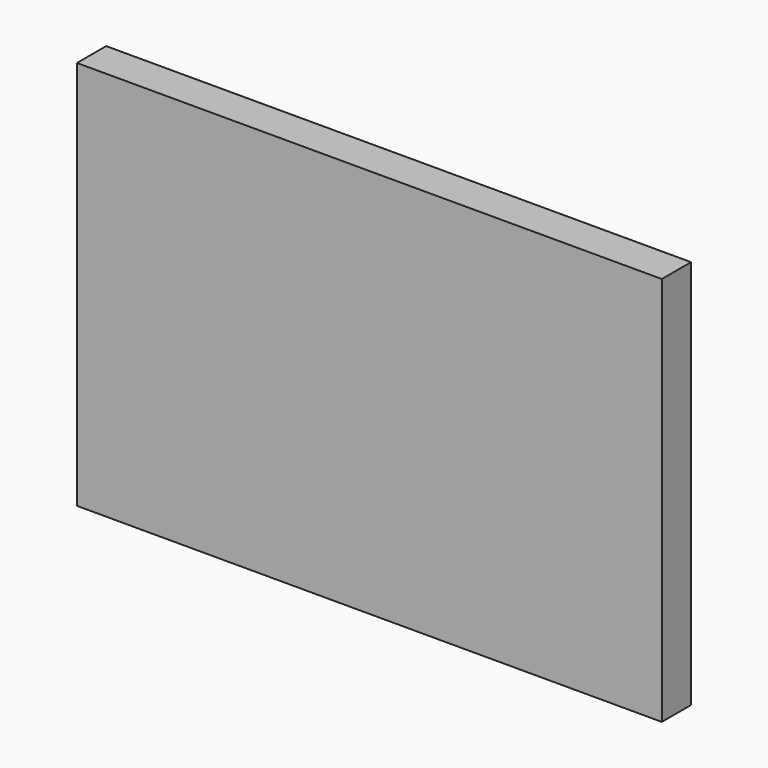
from build123d import *

# Parameters (mm, degrees)
F0_W     = 76.2
F0_H     = 50.8
F1_DEPTH = 4.7625


# Not quite as in the source:
# - a length typed as a fraction of an inch, garbled in the dataset ("3 / 203.2 mm" for 3/8 in), is restored


with BuildPart() as f1:
    # F0 (on Front) → F1 (new body)
    with BuildSketch(Plane.XZ):
        with Locations((38.1, 25.4)):
            Rectangle(F0_W, F0_H)
    extrude(amount=F1_DEPTH)


solid = f1.part
